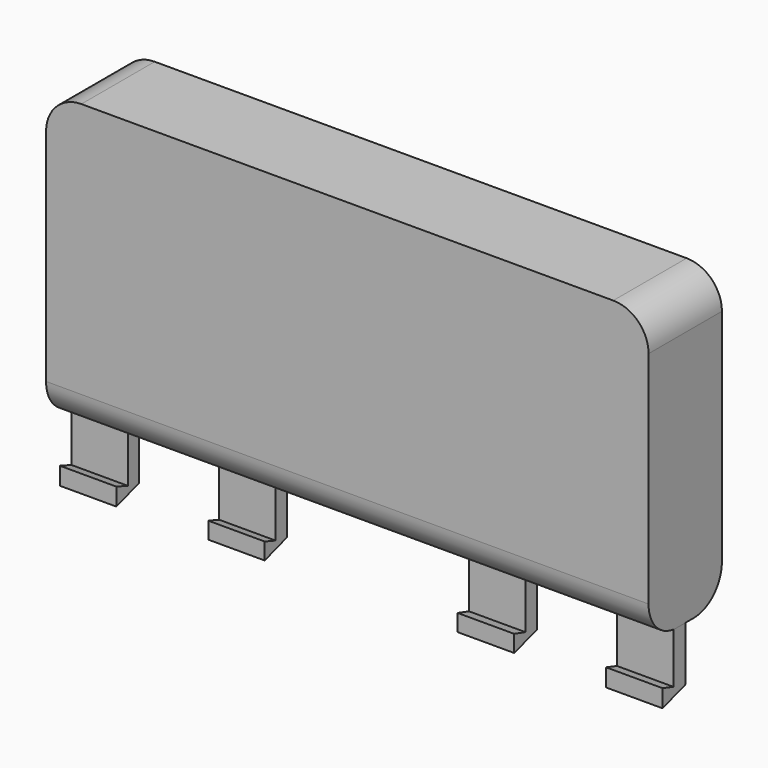
from build123d import *

# Parameters (mm, degrees)
F0_W          = 85.3974372149
F0_H          = 41.2409901619
F1_DEPTH      = 13
F3_DEPTH      = 8
F6_DEPTH      = 8
F9_DEPTH      = 8
F11_DEPTH     = 8
F12_R         = 5
F13_T1_DEPTH  = 110.3974372149
F13_T6_DEPTH  = 110.3974372149
F13_T12_DEPTH = 110.3974372149
F13_T18_DEPTH = 110.3974372149
F13_T25_DEPTH = 110.3974372149
F13_T31_DEPTH = 110.3974372149


# Not quite as in the source:
# - a fillet or chamfer that OpenCascade refuses, or shapes differently, is made with other operations: its cross-section is extruded or revolved along the edge and cut away or added


with BuildPart() as f1:
    # F0 (on Front) → F1 (new body)
    with BuildSketch(Plane.XZ):
        with Locations((42.6987186074, 20.6204950809)):
            Rectangle(F0_W, F0_H)
    extrude(amount=F1_DEPTH)

    # F8 (on offset) → F9 (join)
    with BuildSketch(Plane.YZ.offset(64.3974372149)):
        Polygon((-6.4771878533, 0), (-8.57034605, 0), (-8.57034605, -7.1397153661), (-10.5638308451, -6.5416693687), (-10.5638308451, -8.9338514954), (-6.4771878533, -7.6713105664), align=None)
    extrude(amount=-F9_DEPTH)

    # F12
    f12_edges = [f1.edges().sort_by_distance(p)[0] for p in [
        (0, -6.5, 41.24099),
        (85.397437, -6.5, 41.24099),
    ]]
    fillet(f12_edges, radius=F12_R)

    # F13: fillet of radius 5 on 2 edges, made by hand

    # F13_s2 → F13_t1 (cut)
    with BuildSketch(Plane.YZ.offset(-12.5)):
        with BuildLine():
            ThreePointArc((0, 5), (-1.4644660941, 1.4644660941), (-5, 0))
            Line((-5, 0), (0, 0))
            Line((0, 0), (0, 5))
        make_face()
    extrude(amount=F13_T1_DEPTH, mode=Mode.SUBTRACT)


with BuildPart() as f3:
    # F2 (on face) → F3 (new body)
    with BuildSketch(Plane(origin=(0, 0, 0), x_dir=(0, -1, 0), z_dir=(-1, 0, 0))):
        Polygon((8.5030365735, 0), (6.5, 0), (6.5, -7.7062277123), (10.5613032356, -9.0073291212), (10.5613032356, -6.5101371147), (8.5030365735, -7.2503741831), (8.5030365735, -6.5101371147), align=None)
    extrude(amount=-F3_DEPTH)


with BuildPart() as f6:
    # F5 (on offset) + F3_face (on face) → F6 (new body)
    with BuildSketch(Plane(origin=(21, 0, 0), x_dir=(0, -1, 0), z_dir=(-1, 0, 0))):
        Polygon((8.5787344724, 0), (6.5241577104, 0), (6.5241577104, -7.6201283373), (10.5147780851, -8.9239943773), (10.5147780851, -6.5533285961), (8.5787344724, -7.225017529), align=None)
    with BuildSketch(Plane(origin=(0, -7.9171831416, -4.7191054137), x_dir=(0, -1, 0), z_dir=(-1, 0, 0))):
        Polygon((0.585853432, 4.7191054137), (-1.4171831416, 4.7191054137), (-1.4171831416, -2.9871222987), (2.644120094, -4.2882237076), (2.644120094, -1.791031701), (0.585853432, -2.5312687694), align=None)
    extrude(amount=-F6_DEPTH)


with BuildPart() as f11:
    # F10 (on face) → F11 (new body)
    with BuildSketch(Plane.YZ.offset(85.3974372149)):
        Polygon((-6.4612929709, 0), (-8.5991956294, 0), (-8.5991956294, -7.1200900711), (-10.5256577954, -6.5092607401), (-10.5256577954, -9.0230582282), (-6.4612929709, -7.7074263245), align=None)
    extrude(amount=-F11_DEPTH)


with BuildPart() as f13_tool4:
    # F13_s5 → F13_t6 (new body)
    with BuildSketch(Plane.YZ.offset(-12.5)):
        with BuildLine():
            ThreePointArc((-8, 0), (-11.5355339059, 1.4644660941), (-13, 5))
            Line((-13, 5), (-13, 0))
            Line((-13, 0), (-8, 0))
        make_face()
    extrude(amount=F13_T6_DEPTH)

    split(bisect_by=Plane.YZ.offset(56.3974372149), keep=Keep.BOTTOM)

    split(bisect_by=Plane.XZ.offset(8.57034605), keep=Keep.BOTTOM)


with BuildPart() as f1_1:
    add(f1.part)

    # F13_t3: cut F13_tool4
    add(f13_tool4.part, mode=Mode.SUBTRACT)


with BuildPart() as f13_tool10:
    # F13_s11 → F13_t12 (new body)
    with BuildSketch(Plane.YZ.offset(-12.5)):
        with BuildLine():
            ThreePointArc((-8, 0), (-11.5355339059, 1.4644660941), (-13, 5))
            Line((-13, 5), (-13, 0))
            Line((-13, 0), (-8, 0))
        make_face()
    extrude(amount=F13_T12_DEPTH)

    split(bisect_by=Plane.YZ.offset(56.3974372149), keep=Keep.BOTTOM)

    split(bisect_by=Plane.XZ.offset(8.57034605), keep=Keep.TOP)


with BuildPart() as f1_2:
    add(f1_1.part)

    # F13_t9: cut F13_tool10
    add(f13_tool10.part, mode=Mode.SUBTRACT)


with BuildPart() as f13_tool16:
    # F13_s17 → F13_t18 (new body)
    with BuildSketch(Plane.YZ.offset(-12.5)):
        with BuildLine():
            ThreePointArc((-8, 0), (-11.5355339059, 1.4644660941), (-13, 5))
            Line((-13, 5), (-13, 0))
            Line((-13, 0), (-8, 0))
        make_face()
    extrude(amount=F13_T18_DEPTH)

    split(bisect_by=Plane.YZ.offset(56.3974372149), keep=Keep.TOP)

    split(bisect_by=Plane.XZ.offset(8.57034605), keep=Keep.TOP)

    split(bisect_by=Plane.YZ.offset(64.3974372149), keep=Keep.BOTTOM)


with BuildPart() as f1_3:
    add(f1_2.part)

    # F13_t15: cut F13_tool16
    add(f13_tool16.part, mode=Mode.SUBTRACT)


with BuildPart() as f13_tool23:
    # F13_s24 → F13_t25 (new body)
    with BuildSketch(Plane.YZ.offset(-12.5)):
        with BuildLine():
            ThreePointArc((-8, 0), (-11.5355339059, 1.4644660941), (-13, 5))
            Line((-13, 5), (-13, 0))
            Line((-13, 0), (-8, 0))
        make_face()
    extrude(amount=F13_T25_DEPTH)

    split(bisect_by=Plane.XZ.offset(8.57034605), keep=Keep.BOTTOM)

    split(bisect_by=Plane.YZ.offset(64.3974372149), keep=Keep.TOP)


with BuildPart() as f1_4:
    add(f1_3.part)

    # F13_t22: cut F13_tool23
    add(f13_tool23.part, mode=Mode.SUBTRACT)


with BuildPart() as f13_tool29:
    # F13_s30 → F13_t31 (new body)
    with BuildSketch(Plane.YZ.offset(-12.5)):
        with BuildLine():
            ThreePointArc((-8, 0), (-11.5355339059, 1.4644660941), (-13, 5))
            Line((-13, 5), (-13, 0))
            Line((-13, 0), (-8, 0))
        make_face()
    extrude(amount=F13_T31_DEPTH)

    split(bisect_by=Plane.XZ.offset(8.57034605), keep=Keep.TOP)

    split(bisect_by=Plane.YZ.offset(64.3974372149), keep=Keep.TOP)


with BuildPart() as f1_5:
    add(f1_4.part)

    # F13_t28: cut F13_tool29
    add(f13_tool29.part, mode=Mode.SUBTRACT)


solid = Compound([f3.part, f6.part, f11.part, f1_5.part])
